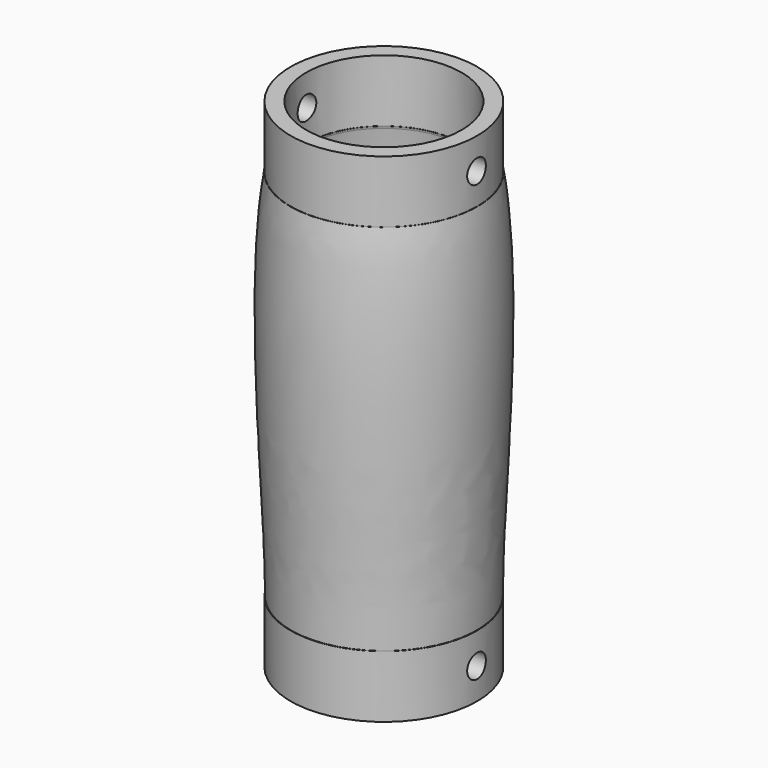
from build123d import *

# Parameters (mm, degrees)
F0_R          = 38.1
F0_R_2        = 31.75
F1_DEPTH      = 25.4
F5_R          = 38.1
F5_R_2        = 31.75
F6_DEPTH      = 25.4
F7_R          = 4.7625
F8_DEPTH      = 41.3056266711
F8_DEPTH_BACK = 41.3056266711


with BuildPart() as f1:
    # F0 (on Top) → F1 (new body)
    with BuildSketch(Plane.XY):
        Circle(F0_R)
        Circle(F0_R_2, mode=Mode.SUBTRACT)
    extrude(amount=F1_DEPTH)

    # F2 (on Front) → F3 (revolve)
    with BuildSketch(Plane.XZ):
        with BuildLine():
            add(Edge.make_bspline(
                [(-37.9096439485, 25.4), (-37.9096439485, 61.3283317127), (-45.343901962, 132.9952478409), (-38.2101392492, 177.8)],
                knots=[0, 0, 0, 0, 152.4002962511, 152.4002962511, 152.4002962511, 152.4002962511], degree=3))
            Line((-37.9096439485, 25.4), (-31.5596439485, 25.4))
            add(Edge.make_bspline(
                [(-31.5596439485, 25.4), (-31.5596439485, 30.0005361538), (-31.7962708065, 40.229659673), (-32.5871723352, 58.0663276532), (-33.5556486353, 77.7063467951), (-34.4446785922, 98.4319215024), (-34.9986327696, 119.5084440497), (-34.9638253583, 140.1883641654), (-34.0922055878, 159.7067304565), (-32.7967181283, 171.41530853), (-31.9391288783, 176.8015367165)],
                knots=[0, 0, 0, 0, 0.125, 0.25, 0.375, 0.5, 0.625, 0.75, 0.875, 1, 1, 1, 1], degree=3))
            Line((-31.9391288783, 176.8015367165), (-31.6526181996, 177.8))
            Line((-31.6526181996, 177.8), (-38.2101392492, 177.8))
        make_face()
    revolve(axis=Axis((0, 0, 43.0460348713), (0, 0, 1)))

    # F5 (on offset) → F6 (join)
    with BuildSketch(Plane.XY.offset(177.8)):
        Circle(F5_R)
        Circle(F5_R_2, mode=Mode.SUBTRACT)
    extrude(amount=F6_DEPTH)

    # F7 (on Right) → F8 (cut, two sides)
    with BuildSketch(Plane.YZ) as f8_sk:
        with Locations((0, 190.5)):
            Circle(F7_R)
        with Locations((0, 12.7)):
            Circle(F7_R)
    extrude(amount=-F8_DEPTH, mode=Mode.SUBTRACT)
    extrude(f8_sk.sketch, amount=F8_DEPTH_BACK, mode=Mode.SUBTRACT)


solid = f1.part
